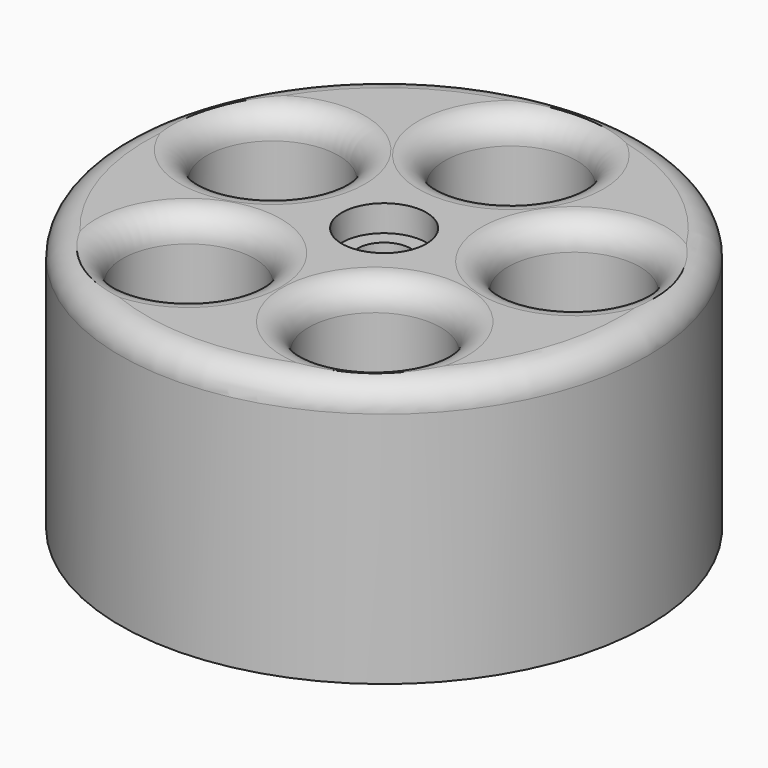
from build123d import *

# Parameters (mm, degrees)
F0_R     = 250
F0_R_2   = 62.5
F0_R_3   = 25
F1_DEPTH = 250
F3_R     = 40
F4_DEPTH = 25


# Not quite as in the source:
# - a fillet or chamfer that OpenCascade refuses, or shapes differently, is made with other operations: its cross-section is extruded or revolved along the edge and cut away or added


with BuildPart() as f1:
    # F0 (on Top) → F1 (new body)
    with BuildSketch(Plane.XY):
        Circle(F0_R)
        with Locations((-88.1677878439, -121.3525491562)):
            Circle(F0_R_2, mode=Mode.SUBTRACT)
        with Locations((88.1677878439, -121.3525491562)):
            Circle(F0_R_2, mode=Mode.SUBTRACT)
        with Locations((-142.6584774443, 46.3525491562)):
            Circle(F0_R_2, mode=Mode.SUBTRACT)
        Circle(F0_R_3, mode=Mode.SUBTRACT)
        with Locations((142.6584774443, 46.3525491562)):
            Circle(F0_R_2, mode=Mode.SUBTRACT)
        with Locations((0, 150)):
            Circle(F0_R_2, mode=Mode.SUBTRACT)
    extrude(amount=F1_DEPTH)

    # F2: fillet of radius 25 on 6 edges, made by hand

    # F2_s1 → F2_t2 (revolve, cut)
    with BuildSketch(Plane.XZ.offset(121.3525491562)):
        with BuildLine():
            ThreePointArc((-25.6677878439, 225), (-18.3454573735, 242.6776695297), (-0.6677878439, 250))
            Line((-0.6677878439, 250), (-25.6677878439, 250))
            Line((-25.6677878439, 250), (-25.6677878439, 225))
        make_face()
    revolve(axis=Axis((-88.1677878439, -121.3525491562, 250), (0, 0, 1)), mode=Mode.SUBTRACT)

    # F2_s3 → F2_t4 (revolve, cut)
    with BuildSketch(Plane.XZ.offset(-46.3525491562)):
        with BuildLine():
            ThreePointArc((-80.1584774443, 225), (-72.8361469739, 242.6776695297), (-55.1584774443, 250))
            Line((-55.1584774443, 250), (-80.1584774443, 250))
            Line((-80.1584774443, 250), (-80.1584774443, 225))
        make_face()
    revolve(axis=Axis((-142.6584774443, 46.3525491562, 250), (0, 0, 1)), mode=Mode.SUBTRACT)

    # F2_s5 → F2_t6 (revolve, cut)
    with BuildSketch(Plane.XZ.offset(-150)):
        with BuildLine():
            ThreePointArc((62.5, 225), (69.8223304703, 242.6776695297), (87.5, 250))
            Line((87.5, 250), (62.5, 250))
            Line((62.5, 250), (62.5, 225))
        make_face()
    revolve(axis=Axis((0, 150, 250), (0, 0, 1)), mode=Mode.SUBTRACT)

    # F2_s7 → F2_t8 (revolve, cut)
    with BuildSketch(Plane.XZ.offset(-46.3525491562)):
        with BuildLine():
            ThreePointArc((205.1584774443, 225), (212.4808079146, 242.6776695297), (230.1584774443, 250))
            Line((230.1584774443, 250), (205.1584774443, 250))
            Line((205.1584774443, 250), (205.1584774443, 225))
        make_face()
    revolve(axis=Axis((142.6584774443, 46.3525491562, 250), (0, 0, 1)), mode=Mode.SUBTRACT)

    # F2_s9 → F2_t10 (revolve, cut)
    with BuildSketch(Plane.XZ.offset(121.3525491562)):
        with BuildLine():
            ThreePointArc((150.6677878439, 225), (157.9901183142, 242.6776695297), (175.6677878439, 250))
            Line((175.6677878439, 250), (150.6677878439, 250))
            Line((150.6677878439, 250), (150.6677878439, 225))
        make_face()
    revolve(axis=Axis((88.1677878439, -121.3525491562, 250), (0, 0, 1)), mode=Mode.SUBTRACT)

    # F2_s11 → F2_t12 (revolve, cut)
    with BuildSketch(Plane.XZ):
        with BuildLine():
            ThreePointArc((250, 225), (242.6776695297, 242.6776695297), (225, 250))
            Line((225, 250), (250, 250))
            Line((250, 250), (250, 225))
        make_face()
    revolve(axis=Axis((0, 0, 250), (0, 0, 1)), mode=Mode.SUBTRACT)

    # F3 (on face) → F4 (cut)
    with BuildSketch(Plane.XY.offset(250)):
        Circle(F3_R)
    extrude(amount=-F4_DEPTH, mode=Mode.SUBTRACT)


solid = f1.part
